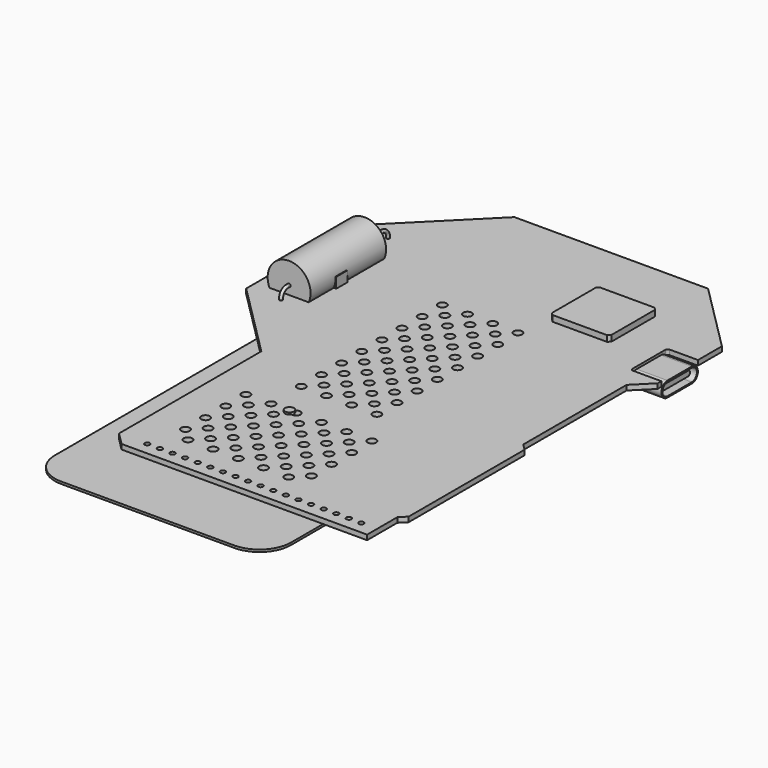
from build123d import *

# Parameters (mm, degrees)
F0_W      = 8.89
F0_H      = 19.939
F1_DEPTH  = 1
F2_R      = 0.8636
F2_R_2    = 0.508
F3_DEPTH  = 1.001
F4_R      = 0.9144
F5_DEPTH  = 0.4064
F6_R      = 0.8128
F7_DEPTH  = 1.524
F9_DEPTH  = 0.45
F11_DEPTH = 6.1976
F13_DEPTH = 5.842
F15_DEPTH = 5.08
F16_R     = 4.3307
F17_DEPTH = 19.05
F20_R     = 0.3175
F24_DEPTH = 4.6482
F25_W     = 12
F25_H     = 12
F26_DEPTH = 1.2
F27_SIZE  = 0.508
F28_DEPTH = 19.939
F29_W     = 3.5052
F29_H     = 2.794
F30_DEPTH = 2.1082


with BuildPart() as f1:
    # F0 (on Top) → F1 (new body)
    with BuildSketch(Plane.XY):
        with BuildLine():
            Line((-2.54, 2.54), (0, 0))
            Line((0, 0), (49.53, 0))
            Line((49.53, 0), (49.53, 7.62))
            Line((49.53, 7.62), (50.8, 8.89))
            Line((50.8, 8.89), (50.8, 38.1))
            Line((50.8, 38.1), (49.53, 39.37))
            Line((49.53, 39.37), (49.53, 65.405))
            Line((49.53, 65.405), (53.0225, 68.8975))
            Line((53.0225, 68.8975), (53.0225, 69.8119))
            Line((53.0225, 69.8119), (47.32528, 69.8119))
            ThreePointArc((47.32528, 69.8119), (46.9714579088, 69.9584579088), (46.8249, 70.31228))
            Line((46.8249, 70.31228), (46.8249, 78.55712))
            ThreePointArc((46.8249, 78.55712), (46.9714579088, 78.9109420912), (47.32528, 79.0575))
            Line((47.32528, 79.0575), (53.0225, 79.0575))
            Line((53.0225, 79.0575), (53.0225, 85.09))
            Line((53.0225, 85.09), (39.0525, 99.06))
            Line((39.0525, 99.06), (0, 99.06))
            Line((0, 99.06), (-17.78, 81.28))
            Line((-17.78, 81.28), (-17.78, 53.6575))
            Line((-17.78, 53.6575), (-2.54, 38.4175))
            Line((-2.54, 38.4175), (-2.54, 2.54))
        make_face()
        with Locations((-11.1125, 65.2145)):
            Rectangle(F0_W, F0_H, mode=Mode.SUBTRACT)
    extrude(amount=F1_DEPTH)

    # F2 (on face) → F3 (cut, through all)
    with BuildSketch(Plane.XY.offset(1)):
        with Locations((17.4625, 50.8)):
            Circle(F2_R)
        with Locations((22.5425, 50.8)):
            Circle(F2_R)
        with Locations((12.3825, 50.8)):
            Circle(F2_R)
        with Locations((9.8425, 53.34)):
            Circle(F2_R)
        with Locations((14.9225, 53.34)):
            Circle(F2_R)
        with Locations((20.0025, 53.34)):
            Circle(F2_R)
        with Locations((25.0825, 53.34)):
            Circle(F2_R)
        with Locations((12.3825, 55.88)):
            Circle(F2_R)
        with Locations((9.8425, 58.42)):
            Circle(F2_R)
        with Locations((14.9225, 58.42)):
            Circle(F2_R)
        with Locations((17.4625, 55.88)):
            Circle(F2_R)
        with Locations((20.0025, 58.42)):
            Circle(F2_R)
        with Locations((22.5425, 55.88)):
            Circle(F2_R)
        with Locations((25.0825, 58.42)):
            Circle(F2_R)
        with Locations((12.3825, 60.96)):
            Circle(F2_R)
        with Locations((9.8425, 63.5)):
            Circle(F2_R)
        with Locations((14.9225, 63.5)):
            Circle(F2_R)
        with Locations((17.4625, 60.96)):
            Circle(F2_R)
        with Locations((20.0025, 63.5)):
            Circle(F2_R)
        with Locations((22.5425, 60.96)):
            Circle(F2_R)
        with Locations((25.0825, 63.5)):
            Circle(F2_R)
        with Locations((12.3825, 66.04)):
            Circle(F2_R)
        with Locations((9.8425, 68.58)):
            Circle(F2_R)
        with Locations((14.9225, 68.58)):
            Circle(F2_R)
        with Locations((17.4625, 66.04)):
            Circle(F2_R)
        with Locations((20.0025, 68.58)):
            Circle(F2_R)
        with Locations((22.5425, 66.04)):
            Circle(F2_R)
        with Locations((25.0825, 68.58)):
            Circle(F2_R)
        with Locations((9.8425, 48.26)):
            Circle(F2_R)
        with Locations((12.3825, 45.72)):
            Circle(F2_R)
        with Locations((14.9225, 48.26)):
            Circle(F2_R)
        with Locations((17.4625, 45.72)):
            Circle(F2_R)
        with Locations((20.0025, 48.26)):
            Circle(F2_R)
        with Locations((22.5425, 45.72)):
            Circle(F2_R)
        with Locations((25.0825, 48.26)):
            Circle(F2_R)
        with Locations((9.8425, 43.18)):
            Circle(F2_R)
        with Locations((12.3825, 40.64)):
            Circle(F2_R)
        with Locations((14.9225, 43.18)):
            Circle(F2_R)
        with Locations((17.4625, 40.64)):
            Circle(F2_R)
        with Locations((20.0025, 43.18)):
            Circle(F2_R)
        with Locations((22.5425, 40.64)):
            Circle(F2_R)
        with Locations((25.0825, 43.18)):
            Circle(F2_R)
        with Locations((9.8425, 38.1)):
            Circle(F2_R)
        with Locations((12.3825, 35.56)):
            Circle(F2_R)
        with Locations((14.9225, 38.1)):
            Circle(F2_R)
        with Locations((17.4625, 35.56)):
            Circle(F2_R)
        with Locations((20.0025, 38.1)):
            Circle(F2_R)
        with Locations((22.5425, 35.56)):
            Circle(F2_R)
        with Locations((25.0825, 38.1)):
            Circle(F2_R)
        with Locations((9.8425, 33.02)):
            Circle(F2_R)
        with Locations((14.9225, 33.02)):
            Circle(F2_R)
        with Locations((20.0025, 33.02)):
            Circle(F2_R)
        with Locations((25.0825, 33.02)):
            Circle(F2_R)
        with Locations((4.7625, 25.4)):
            Circle(F2_R)
        with Locations((9.8425, 25.4)):
            Circle(F2_R)
        with Locations((14.9225, 25.4)):
            Circle(F2_R)
        with Locations((20.0025, 25.4)):
            Circle(F2_R)
        with Locations((25.0825, 25.4)):
            Circle(F2_R)
        with Locations((30.1625, 25.4)):
            Circle(F2_R)
        with Locations((7.3025, 22.86)):
            Circle(F2_R)
        with Locations((12.3825, 22.86)):
            Circle(F2_R)
        with Locations((17.4625, 22.86)):
            Circle(F2_R)
        with Locations((22.5425, 22.86)):
            Circle(F2_R)
        with Locations((27.6225, 22.86)):
            Circle(F2_R)
        with Locations((4.7625, 20.32)):
            Circle(F2_R)
        with Locations((9.8425, 20.32)):
            Circle(F2_R)
        with Locations((14.9225, 20.32)):
            Circle(F2_R)
        with Locations((20.0025, 20.32)):
            Circle(F2_R)
        with Locations((25.0825, 20.32)):
            Circle(F2_R)
        with Locations((30.1625, 20.32)):
            Circle(F2_R)
        with Locations((27.6225, 17.78)):
            Circle(F2_R)
        with Locations((22.5425, 17.78)):
            Circle(F2_R)
        with Locations((17.4625, 17.78)):
            Circle(F2_R)
        with Locations((12.3825, 17.78)):
            Circle(F2_R)
        with Locations((7.3025, 17.78)):
            Circle(F2_R)
        with Locations((4.7625, 15.24)):
            Circle(F2_R)
        with Locations((9.8425, 15.24)):
            Circle(F2_R)
        with Locations((14.9225, 15.24)):
            Circle(F2_R)
        with Locations((20.0025, 15.24)):
            Circle(F2_R)
        with Locations((25.0825, 15.24)):
            Circle(F2_R)
        with Locations((30.1625, 15.24)):
            Circle(F2_R)
        with Locations((27.6225, 12.7)):
            Circle(F2_R)
        with Locations((22.5425, 12.7)):
            Circle(F2_R)
        with Locations((17.4625, 12.7)):
            Circle(F2_R)
        with Locations((12.3825, 12.7)):
            Circle(F2_R)
        with Locations((7.3025, 12.7)):
            Circle(F2_R)
        with Locations((4.7625, 10.16)):
            Circle(F2_R)
        with Locations((9.8425, 10.16)):
            Circle(F2_R)
        with Locations((14.9225, 10.16)):
            Circle(F2_R)
        with Locations((20.0025, 10.16)):
            Circle(F2_R)
        with Locations((25.0825, 10.16)):
            Circle(F2_R)
        with Locations((30.1625, 10.16)):
            Circle(F2_R)
        with Locations((27.6225, 7.62)):
            Circle(F2_R)
        with Locations((22.5425, 7.62)):
            Circle(F2_R)
        with Locations((17.4625, 7.62)):
            Circle(F2_R)
        with Locations((12.3825, 7.62)):
            Circle(F2_R)
        with Locations((7.3025, 7.62)):
            Circle(F2_R)
        with Locations((3.175, 2.54)):
            Circle(F2_R_2)
        with Locations((5.715, 2.54)):
            Circle(F2_R_2)
        with Locations((8.255, 2.54)):
            Circle(F2_R_2)
        with Locations((10.795, 2.54)):
            Circle(F2_R_2)
        with Locations((13.335, 2.54)):
            Circle(F2_R_2)
        with Locations((15.875, 2.54)):
            Circle(F2_R_2)
        with Locations((18.415, 2.54)):
            Circle(F2_R_2)
        with Locations((20.955, 2.54)):
            Circle(F2_R_2)
        with Locations((23.495, 2.54)):
            Circle(F2_R_2)
        with Locations((26.035, 2.54)):
            Circle(F2_R_2)
        with Locations((28.575, 2.54)):
            Circle(F2_R_2)
        with Locations((31.115, 2.54)):
            Circle(F2_R_2)
        with Locations((33.655, 2.54)):
            Circle(F2_R_2)
        with Locations((36.195, 2.54)):
            Circle(F2_R_2)
        with Locations((38.735, 2.54)):
            Circle(F2_R_2)
        with Locations((41.275, 2.54)):
            Circle(F2_R_2)
        with Locations((43.815, 2.54)):
            Circle(F2_R_2)
        with Locations((46.355, 2.54)):
            Circle(F2_R_2)
    extrude(amount=-F3_DEPTH, mode=Mode.SUBTRACT)

    # F28 (add, through all): a face of the model
    f28_faces = [f1.faces().sort_by_distance(p)[0] for p in [
        (-11.1125, 75.184, 0.5),
    ]]
    extrude(f28_faces, amount=F28_DEPTH)


with BuildPart() as f5:
    # F4 (on face) → F5 (new body)
    with BuildSketch(Plane.XY.offset(1)):
        with Locations((13.8691896573, 25.0180773437)):
            Circle(F4_R)
    extrude(amount=F5_DEPTH)

    # F6 (on face) → F7 (join)
    with BuildSketch(Plane(origin=(0, 0, 1), x_dir=(1, 0, 0), z_dir=(0, 0, -1))):
        with Locations((13.8691896573, -25.0180773437)):
            Circle(F6_R)
    extrude(amount=F7_DEPTH)


with BuildPart() as f9:
    # F8 (on face) → F9 (new body)
    with BuildSketch(Plane(origin=(0, 0, -0.524), x_dir=(1, 0, 0), z_dir=(0, 0, -1))):
        with BuildLine():
            ThreePointArc((40.0282551781, 7.313141322), (38.1683832386, 11.8032693825), (33.6782551781, 13.663141322))
            Line((33.6782551781, 13.663141322), (-1.2467448219, 13.663141322))
            ThreePointArc((-1.2467448219, 13.663141322), (-5.7368728825, 11.8032693825), (-7.5967448219, 7.313141322))
            Line((-7.5967448219, 7.313141322), (-7.5967448219, -65.2976975123))
            ThreePointArc((-7.5967448219, -65.2976975123), (-7.890509229, -67.2067576063), (-8.7446221267, -68.939183399))
            Line((-8.7446221267, -68.939183399), (-12.0051175172, -73.597033957))
            ThreePointArc((-12.0051175172, -73.597033957), (-12.8592304149, -75.3294597497), (-13.1529948219, -77.2385198437))
            Line((-13.1529948219, -77.2385198437), (-13.1529948219, -87.936858678))
            Line((-13.1529948219, -87.936858678), (45.5845051781, -87.936858678))
            Line((45.5845051781, -87.936858678), (45.5845051781, -77.2385198437))
            ThreePointArc((45.5845051781, -77.2385198437), (45.290740771, -75.3294597497), (44.4366278733, -73.597033957))
            Line((44.4366278733, -73.597033957), (41.1761324828, -68.939183399))
            ThreePointArc((41.1761324828, -68.939183399), (40.3220195851, -67.2067576063), (40.0282551781, -65.2976975123))
            Line((40.0282551781, -65.2976975123), (40.0282551781, 7.313141322))
        make_face()
    extrude(amount=F9_DEPTH)


with BuildPart() as f11:
    # F10 (on face) → F11 (new body, through all)
    with BuildSketch(Plane.YZ.offset(53.0225)):
        with BuildLine():
            Line((77.5081, 0.5), (71.3613, 0.5))
            ThreePointArc((71.3613, 0.5), (69.8373, -1.024), (71.3613, -2.548))
            Line((71.3613, -2.548), (77.5081, -2.548))
            ThreePointArc((77.5081, -2.548), (79.0321, -1.024), (77.5081, 0.5))
        make_face()
    extrude(amount=-F11_DEPTH)

    # F12 (on face) → F13 (cut)
    with BuildSketch(Plane.YZ.offset(53.0225)):
        with BuildLine():
            Line((71.3613, -2.294), (77.5081, -2.294))
            ThreePointArc((77.5081, -2.294), (78.7781, -1.024), (77.5081, 0.246))
            Line((77.5081, 0.246), (71.3613, 0.246))
            ThreePointArc((71.3613, 0.246), (70.0913, -1.024), (71.3613, -2.294))
        make_face()
    extrude(amount=-F13_DEPTH, mode=Mode.SUBTRACT)

    # F14 (on face) → F15 (join)
    with BuildSketch(Plane.YZ.offset(47.1805)):
        with BuildLine():
            Line((77.5081, -0.516), (71.3613, -0.516))
            ThreePointArc((71.3613, -0.516), (70.8533, -1.024), (71.3613, -1.532))
            Line((71.3613, -1.532), (77.5081, -1.532))
            ThreePointArc((77.5081, -1.532), (78.0161, -1.024), (77.5081, -0.516))
        make_face()
    extrude(amount=F15_DEPTH)

    # F23 (on face) → F24 (join)
    with BuildSketch(Plane(origin=(46.8249, 0, 0), x_dir=(0, -1, 0), z_dir=(-1, 0, 0))):
        with BuildLine():
            Line((-77.5081, -2.548), (-71.3613, -2.548))
            ThreePointArc((-71.3613, -2.548), (-70.0124667264, -1.7333833942), (-70.1056045592, -0.1604))
            Line((-70.1056045592, -0.1604), (-78.7637954408, -0.1604))
            ThreePointArc((-78.7637954408, -0.1604), (-78.8569332736, -1.7333833942), (-77.5081, -2.548))
        make_face()
    extrude(amount=F24_DEPTH)


with BuildPart() as f17:
    # F16 (on face) → F17 (new body)
    with BuildSketch(Plane.XZ.offset(-75.184)):
        with Locations((-11.1125, 2.74879)):
            Circle(F16_R)
    extrude(amount=F17_DEPTH)

    # F21: sweep along a path in F19
    with BuildLine(Plane.YZ.offset(-11.1125)) as f21_path:
        Line((81.0768, 0.99873), (81.0768, 1.22479))
        ThreePointArc((81.0768, 1.22479), (80.6304307345, 2.3024207345), (79.5528, 2.74879))
        Line((79.5528, 2.74879), (75.184, 2.74879))
    # F20 (on face) → F21 (sweep)
    with BuildSketch(Plane(origin=(0, 75.184, 0), x_dir=(-1, 0, 0), z_dir=(0, 1, 0))):
        with Locations((11.1125, 2.74879)):
            Circle(F20_R)
    sweep(path=f21_path.line)

    # F22: sweep along a path in F19
    with BuildLine(Plane.YZ.offset(-11.1125)) as f22_path:
        Line((75.184, 2.74879), (56.134, 2.74879))
        Line((56.134, 2.74879), (55.626, 2.74879))
        ThreePointArc((55.626, 2.74879), (54.5483692655, 2.3024207345), (54.102, 1.22479))
        Line((54.102, 1.22479), (54.102, 0.99873))
    # F20 (on face) → F22 (sweep)
    with BuildSketch(Plane(origin=(0, 75.184, 0), x_dir=(-1, 0, 0), z_dir=(0, 1, 0))):
        with Locations((11.1125, 2.74879)):
            Circle(F20_R)
    sweep(path=f22_path.line)


with BuildPart() as f26:
    # F25 (on face) → F26 (new body)
    with BuildSketch(Plane.XY.offset(1)):
        with Locations((32.4677838366, 80.9408314526)):
            Rectangle(F25_W, F25_H)
    extrude(amount=F26_DEPTH)

    # F27
    f27_edges = [f26.edges().sort_by_distance(p)[0] for p in [
        (38.467784, 74.940831, 1.6),
        (26.467784, 74.940831, 1.6),
        (26.467784, 86.940831, 1.6),
        (38.467784, 86.940831, 1.6),
    ]]
    chamfer(f27_edges, length=F27_SIZE)


with BuildPart() as f30:
    # F29 (on face) → F30 (new body)
    with BuildSketch(Plane.XY.offset(1)):
        with Locations((-8.4085476119, 63.8421217538)):
            Rectangle(F29_W, F29_H)
    extrude(amount=F30_DEPTH)


solid = Compound([f1.part, f5.part, f9.part, f11.part, f17.part, f26.part, f30.part])
